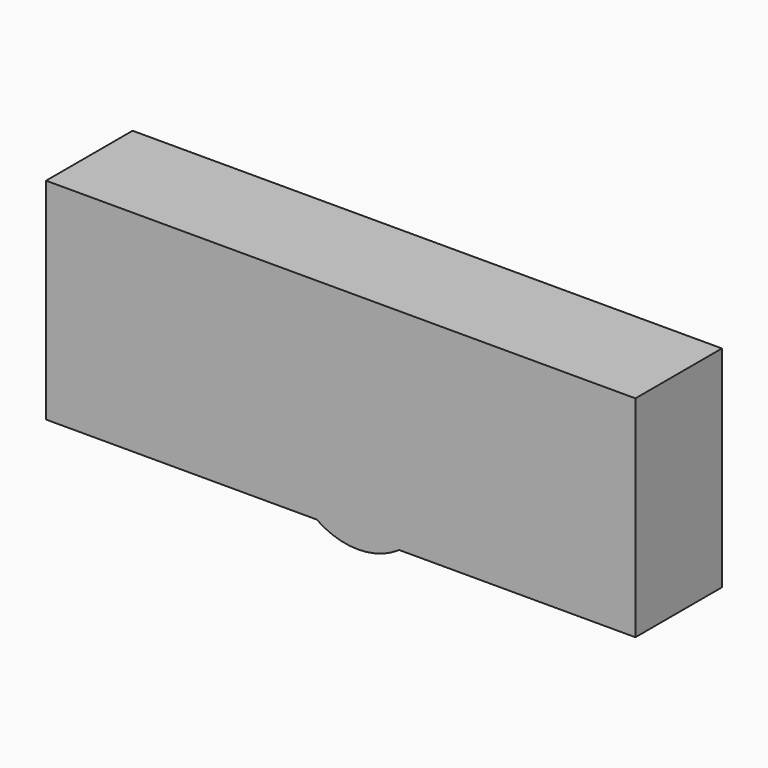
from build123d import *

# Parameters (mm, degrees)
F0_W     = 138.4305804968
F0_H     = 49.4050085545
F1_DEPTH = 25.4
F2_R     = 17.004974152
F3_DEPTH = 25.4


# Not quite as in the source:
# - the program builds the solid bodies; features that only make, move or delete a surface that nothing else refers to are left out


with BuildPart() as f1:
    # F0 (on Front) → F1 (new body)
    with BuildSketch(Plane.XZ):
        with Locations((52.0747005939, 24.7025042772)):
            Rectangle(F0_W, F0_H)
    extrude(amount=F1_DEPTH)

    # F2 (on Front) → F3 (join)
    with BuildSketch(Plane.XZ):
        with Locations((56.1164021492, 13.9775313437)):
            Circle(F2_R)
    extrude(amount=F3_DEPTH)


solid = f1.part
